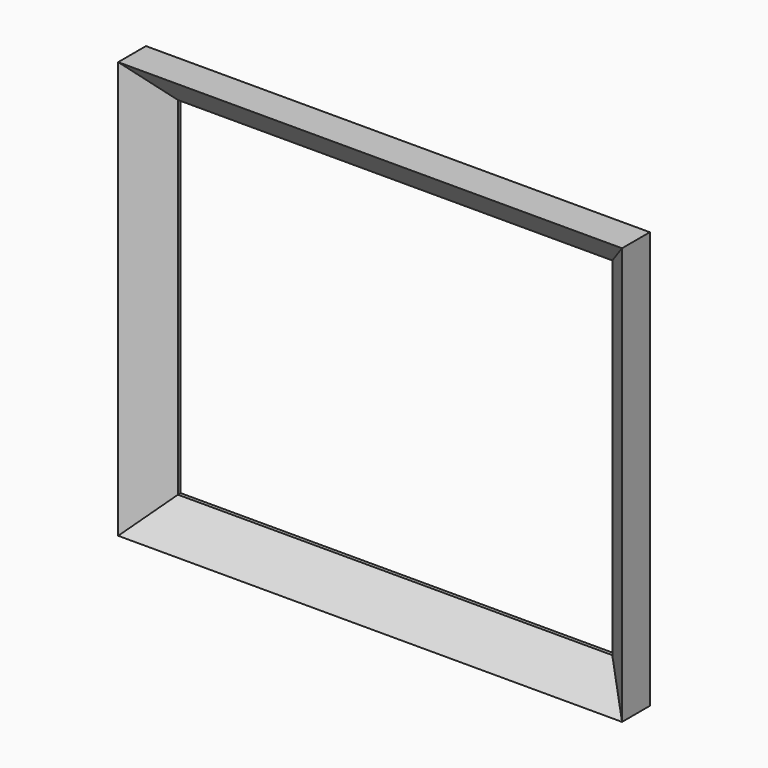
from build123d import *

# Parameters (mm, degrees)
F1_W     = 58
F1_H     = 48
F1_W_2   = 50
F1_H_2   = 40
F2_DEPTH = 4
F3_SIZE2 = 3.59999
F3_SIZE  = 3.99999


# Not quite as in the source:
# - a fillet or chamfer is up to 0.001 mm smaller than in the source, because OpenCascade refuses the exact size


with BuildPart() as f2:
    # F1 (on Front) → F2 (new body)
    with BuildSketch(Plane.XZ):
        Rectangle(F1_W, F1_H)
        Rectangle(F1_W_2, F1_H_2, mode=Mode.SUBTRACT)
    extrude(amount=F2_DEPTH)

    # F3 (size 4 and 3.6 in the source; OpenCascade refuses exactly that, so slightly less here)
    f3_edges = [f2.edges().sort_by_distance(p)[0] for p in [
        (-25, -4, 0),
        (0, -4, 20),
        (25, -4, 0),
        (0, -4, -20),
    ]]
    f3_side = f2.faces().sort_by_distance((28.247139, -4, 0))[0]
    chamfer(f3_edges, length=F3_SIZE, length2=F3_SIZE2, reference=f3_side)


solid = f2.part
